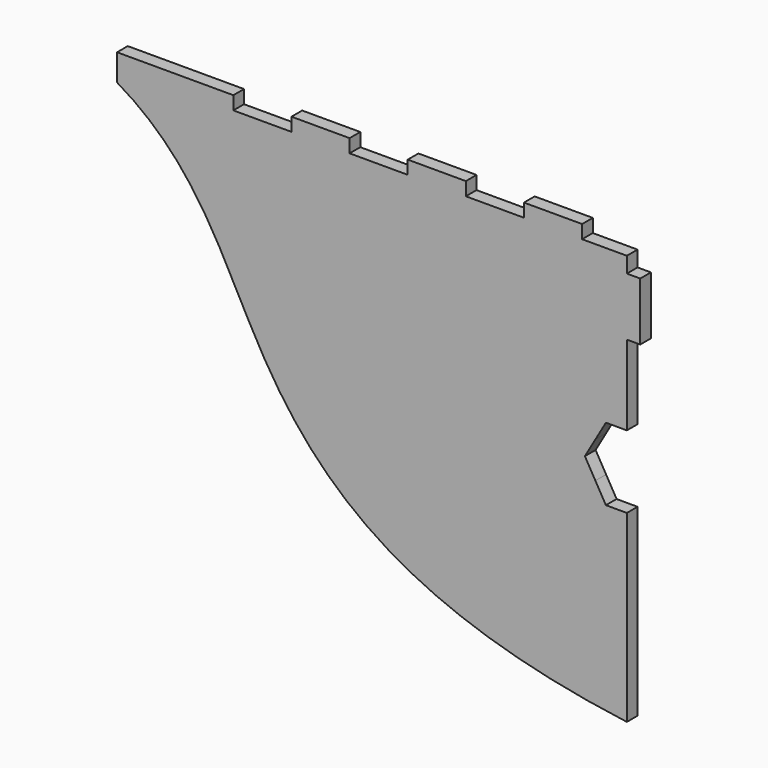
from build123d import *

# Parameters (mm, degrees)
F0_W      = 279.4
F0_H      = 330.2
F1_DEPTH  = 5.842
F2_W      = 25.4
F2_H      = 5.842
F2_W_2    = 76.2
F2_W_3    = 5.842
F2_H_2    = 25.4
F2_H_3    = 38.1
F3_DEPTH  = 5.842
F5_W      = 5.842
F5_H      = 12.7
F6_DEPTH  = 5.842
F7_DEPTH  = 5.842
F8_W      = 5.842
F8_H      = 25.4
F8_H_2    = 48.641
F8_H_3    = 34.925
F8_H_4    = 11.684
F9_DEPTH  = 5.842
F10_W     = 246.7240431406
F10_H     = 1.016
F11_DEPTH = 5.842
F13_W     = 25.4
F13_H     = 5.842
F13_W_2   = 19.558
F14_DEPTH = 5.842


# Not quite as in the source:
# - a feature names something its author has since deleted; it is built from what else it names


with BuildPart() as f1:
    # F0 (on Front) → F1 (new body)
    with BuildSketch(Plane.XZ):
        with Locations((25.751306051, 40.8756073241)):
            Rectangle(F0_W, F0_H)
    extrude(amount=F1_DEPTH)

    # F2 (on face) → F3 (cut, through all)
    with BuildSketch(Plane.XZ.offset(5.842)):
        with Locations((152.751306051, -121.3033926759)):
            Rectangle(F2_W, F2_H)
        with Locations((101.951306051, -121.3033926759)):
            Rectangle(F2_W, F2_H)
        with Locations((51.151306051, -121.3033926759)):
            Rectangle(F2_W, F2_H)
        with Locations((0.351306051, -121.3033926759)):
            Rectangle(F2_W, F2_H)
        with Locations((-75.848693949, -121.3033926759)):
            Rectangle(F2_W_2, F2_H)
        with Locations((162.530306051, -86.1243926759)):
            Rectangle(F2_W_3, F2_H_2)
        with Locations((162.530306051, -28.9743926759)):
            Rectangle(F2_W_3, F2_H_3)
        with Locations((-111.027693949, -86.1243926759)):
            Rectangle(F2_W_3, F2_H_2)
        with Locations((-111.027693949, -35.3243926759)):
            Rectangle(F2_W_3, F2_H_2)
        with Locations((-111.027693949, 15.4756073241)):
            Rectangle(F2_W_3, F2_H_2)
        with Locations((-111.027693949, 66.2756073241)):
            Rectangle(F2_W_3, F2_H_2)
        with Locations((-111.027693949, 167.8756073241)):
            Rectangle(F2_W_3, F2_H_2)
        with Locations((-111.027693949, 117.0756073241)):
            Rectangle(F2_W_3, F2_H_2)
    extrude(amount=-F3_DEPTH, mode=Mode.SUBTRACT)

    # F5 (on face) → F6 (cut, through all)
    with BuildSketch(Plane.XZ.offset(5.842)):
        with Locations((162.530306051, 2.7756073241)):
            Rectangle(F5_W, F5_H)
    extrude(amount=-F6_DEPTH, mode=Mode.SUBTRACT)

    # F4 (on face) → F7 (cut, through all)
    with BuildSketch(Plane.XZ.offset(5.842)):
        with BuildLine():
            Line((165.451306051, 15.4756073241), (159.609306051, 15.4756073241))
            add(Edge.make_bspline(
                [(159.609306051, 15.4756073241), (73.376306051, 28.1756073241), (-24.3765935073, 60.3637718481), (-21.873693949, 193.2756073241), (-113.948693949, 205.9756073241)],
                knots=[0, 0, 0, 0, 0.507272, 1, 1, 1, 1], degree=3))
            Line((-113.948693949, 205.9756073241), (-113.948693949, 180.5756073241))
            Line((-113.948693949, 180.5756073241), (-108.106693949, 180.5756073241))
            Line((-108.106693949, 180.5756073241), (-108.106693949, 155.1756073241))
            Line((-108.106693949, 155.1756073241), (-113.948693949, 155.1756073241))
            Line((-113.948693949, 155.1756073241), (-113.948693949, 129.7756073241))
            Line((-113.948693949, 129.7756073241), (-108.106693949, 129.7756073241))
            Line((-108.106693949, 129.7756073241), (-108.106693949, 104.3756073241))
            Line((-108.106693949, 104.3756073241), (-113.948693949, 104.3756073241))
            Line((-113.948693949, 104.3756073241), (-113.948693949, 78.9756073241))
            Line((-113.948693949, 78.9756073241), (-108.106693949, 78.9756073241))
            Line((-108.106693949, 78.9756073241), (-108.106693949, 53.5756073241))
            Line((-108.106693949, 53.5756073241), (-113.948693949, 53.5756073241))
            Line((-113.948693949, 53.5756073241), (-113.948693949, 28.1756073241))
            Line((-113.948693949, 28.1756073241), (-108.106693949, 28.1756073241))
            Line((-108.106693949, 28.1756073241), (-108.106693949, 2.7756073241))
            Line((-108.106693949, 2.7756073241), (-113.948693949, 2.7756073241))
            Line((-113.948693949, 2.7756073241), (-113.948693949, -22.6243926759))
            Line((-113.948693949, -22.6243926759), (-108.106693949, -22.6243926759))
            Line((-108.106693949, -22.6243926759), (-108.106693949, -48.0243926759))
            Line((-108.106693949, -48.0243926759), (-113.948693949, -48.0243926759))
            Line((-113.948693949, -48.0243926759), (-113.948693949, -73.4243926759))
            Line((-113.948693949, -73.4243926759), (-108.106693949, -73.4243926759))
            Line((-108.106693949, -73.4243926759), (-108.106693949, -98.8243926759))
            Line((-108.106693949, -98.8243926759), (-113.948693949, -98.8243926759))
            Line((-113.948693949, -98.8243926759), (-113.948693949, -118.3823926759))
            Line((-113.948693949, -118.3823926759), (-37.748693949, -118.3823926759))
            Line((-37.748693949, -118.3823926759), (-37.748693949, -124.2243926759))
            Line((-37.748693949, -124.2243926759), (-12.348693949, -124.2243926759))
            Line((-12.348693949, -124.2243926759), (-12.348693949, -118.3823926759))
            Line((-12.348693949, -118.3823926759), (13.051306051, -118.3823926759))
            Line((13.051306051, -118.3823926759), (13.051306051, -124.2243926759))
            Line((13.051306051, -124.2243926759), (38.451306051, -124.2243926759))
            Line((38.451306051, -124.2243926759), (38.451306051, -118.3823926759))
            Line((38.451306051, -118.3823926759), (63.851306051, -118.3823926759))
            Line((63.851306051, -118.3823926759), (63.851306051, -124.2243926759))
            Line((63.851306051, -124.2243926759), (89.251306051, -124.2243926759))
            Line((89.251306051, -124.2243926759), (89.251306051, -118.3823926759))
            Line((89.251306051, -118.3823926759), (114.651306051, -118.3823926759))
            Line((114.651306051, -118.3823926759), (114.651306051, -124.2243926759))
            Line((114.651306051, -124.2243926759), (140.051306051, -124.2243926759))
            Line((140.051306051, -124.2243926759), (140.051306051, -118.3823926759))
            Line((140.051306051, -118.3823926759), (165.451306051, -118.3823926759))
            Line((165.451306051, -118.3823926759), (165.451306051, -98.8243926759))
            Line((165.451306051, -98.8243926759), (159.609306051, -98.8243926759))
            Line((159.609306051, -98.8243926759), (159.609306051, -73.4243926759))
            Line((159.609306051, -73.4243926759), (165.451306051, -73.4243926759))
            Line((165.451306051, -73.4243926759), (165.451306051, -48.0243926759))
            Line((165.451306051, -48.0243926759), (159.609306051, -48.0243926759))
            Line((159.609306051, -48.0243926759), (159.609306051, -9.9243926759))
            Line((159.609306051, -9.9243926759), (165.451306051, -9.9243926759))
            Line((165.451306051, -9.9243926759), (165.451306051, 15.4756073241))
        make_face()
        with BuildLine():
            add(Edge.make_bspline(
                [(159.609306051, 15.4756073241), (73.376306051, 28.1756073241), (-24.3765935073, 60.3637718481), (-21.873693949, 193.2756073241), (-113.948693949, 205.9756073241)],
                knots=[0, 0, 0, 0, 0.507272, 1, 1, 1, 1], degree=3))
            Line((159.609306051, 15.4756073241), (159.609306051, 21.8256073241))
            add(Edge.make_bspline(
                [(159.609306051, 21.8256073241), (63.851306051, 34.5256073241), (-5.6173037023, 95.4914607938), (-31.4644745687, 187.7697107475), (-87.114737086, 205.9756073241)],
                knots=[0, 0, 0, 0, 0.5236819738, 0.940243193, 0.940243193, 0.940243193, 0.940243193], degree=3))
            Line((-87.114737086, 205.9756073241), (-113.948693949, 205.9756073241))
        make_face()
    extrude(amount=-F7_DEPTH, mode=Mode.SUBTRACT)

    # F8 (on face) → F9 (cut, through all)
    with BuildSketch(Plane.XZ.offset(5.842)):
        Polygon((165.451306051, 15.4756073241), (165.451306051, 28.1756073241), (159.609306051, 28.1756073241), (159.609306051, 21.8256073241), (159.609306051, 15.4756073241), align=None)
        with Locations((162.530306051, 40.8756073241)):
            Rectangle(F8_W, F8_H)
        with Locations((162.530306051, 77.8961073241)):
            Rectangle(F8_W, F8_H_2)
        with BuildLine():
            Line((159.609306051, 102.2166073241), (165.451306051, 102.2166073241))
            Line((165.451306051, 102.2166073241), (165.451306051, 103.3306229057))
            ThreePointArc((165.451306051, 103.3306229057), (162.5829399691, 102.4975980153), (159.609306051, 102.2166073241))
        make_face()
        with BuildLine():
            ThreePointArc((145.861152343, 110.1541080567), (151.6718056847, 104.3434542505), (159.609306051, 102.2166073241))
            Line((159.609306051, 102.2166073241), (159.609306051, 133.9666073241))
            ThreePointArc((159.609306051, 133.9666073241), (151.6718056847, 131.8397603977), (145.861152343, 126.0291065915))
            ThreePointArc((145.861152343, 126.0291065915), (143.734306051, 118.0916073241), (145.861152343, 110.1541080567))
        make_face()
        with BuildLine():
            Line((150.4438705276, 102.2166073241), (159.609306051, 102.2166073241))
            ThreePointArc((159.609306051, 102.2166073241), (151.6718056847, 104.3434542505), (145.861152343, 110.1541080567))
            Line((145.861152343, 110.1541080567), (150.4438705276, 102.2166073241))
        make_face()
        with BuildLine():
            Line((159.609306051, 133.9666073241), (159.609306051, 102.2166073241))
            ThreePointArc((159.609306051, 102.2166073241), (162.5829399691, 102.4975980153), (165.451306051, 103.3306229057))
            Line((165.451306051, 103.3306229057), (165.451306051, 132.8525917425))
            ThreePointArc((165.451306051, 132.8525917425), (162.5829399691, 133.6856166328), (159.609306051, 133.9666073241))
        make_face()
        with BuildLine():
            Line((165.451306051, 133.9666073241), (159.609306051, 133.9666073241))
            ThreePointArc((159.609306051, 133.9666073241), (162.5829399691, 133.6856166328), (165.451306051, 132.8525917425))
            Line((165.451306051, 132.8525917425), (165.451306051, 133.9666073241))
        make_face()
        with BuildLine():
            ThreePointArc((145.861152343, 126.0291065915), (151.6718056847, 131.8397603977), (159.609306051, 133.9666073241))
            Line((159.609306051, 133.9666073241), (150.4438705276, 133.9666073241))
            Line((150.4438705276, 133.9666073241), (145.861152343, 126.0291065915))
        make_face()
        with Locations((162.530306051, 151.4291073241)):
            Rectangle(F8_W, F8_H_3)
        with BuildLine():
            Line((141.2784350042, 118.0916073241), (145.861152343, 110.1541080567))
            ThreePointArc((145.861152343, 110.1541080567), (143.734306051, 118.0916073241), (145.861152343, 126.0291065915))
            Line((145.861152343, 126.0291065915), (141.2784350042, 118.0916073241))
        make_face()
        with Locations((162.530306051, 200.1336073241)):
            Rectangle(F8_W, F8_H_4)
    extrude(amount=-F9_DEPTH, mode=Mode.SUBTRACT)

    # F10 (on face) → F11 (join, through all)
    with BuildSketch(Plane.XZ.offset(5.842)):
        with Locations((36.2472844807, 206.4836073241)):
            Rectangle(F10_W, F10_H)
    extrude(amount=-F11_DEPTH)

    # F13 (on face) → F14 (cut, through all)
    with BuildSketch(Plane.XZ.offset(5.842)):
        with Locations((51.151306051, 204.0706073241)):
            Rectangle(F13_W, F13_H)
        with Locations((101.951306051, 204.0706073241)):
            Rectangle(F13_W, F13_H)
        with Locations((149.830306051, 204.0706073241)):
            Rectangle(F13_W_2, F13_H)
        with BuildLine():
            add(Edge.make_bspline(
                [(-64.0656111495, 195.8912068503), (-64.4986133811, 197.8821506555), (-64.5462177809, 200.9608220943), (-64.8897370896, 206.9916073241)],
                knots=[0.7783755915, 0.7783755915, 0.7783755915, 0.7783755915, 1, 1, 1, 1], degree=3))
            Line((-64.8897370896, 206.9916073241), (-87.1147370896, 206.9916073241))
            Line((-87.1147370896, 206.9916073241), (-87.1147370896, 205.9756073241))
            add(Edge.make_bspline(
                [(-64.0656111419, 195.8912068549), (-70.8038372609, 199.7329606353), (-78.4197996839, 203.1310721158), (-87.114737086, 205.9756073241)],
                knots=[0.8751586172, 0.8751586172, 0.8751586172, 0.8751586172, 0.940243193, 0.940243193, 0.940243193, 0.940243193], degree=3))
        make_face()
        with Locations((0.351306051, 204.0706073241)):
            Rectangle(F13_W, F13_H)
        with BuildLine():
            Line((-63.148693949, 195.362557311), (-63.148693949, 206.9916073241))
            Line((-63.148693949, 206.9916073241), (-64.8897370896, 206.9916073241))
            add(Edge.make_bspline(
                [(-64.0656111495, 195.8912068503), (-64.4986133811, 197.8821506555), (-64.5462177809, 200.9608220943), (-64.8897370896, 206.9916073241)],
                knots=[0.7783755915, 0.7783755915, 0.7783755915, 0.7783755915, 1, 1, 1, 1], degree=3))
            add(Edge.make_bspline(
                [(-63.148693949, 195.362557311), (-63.4525182871, 195.5396905387), (-63.7581509788, 195.7159105346), (-64.0656111419, 195.8912068549)],
                knots=[0.8721888572, 0.8721888572, 0.8721888572, 0.8721888572, 0.8751586172, 0.8751586172, 0.8751586172, 0.8751586172], degree=3))
        make_face()
    extrude(amount=-F14_DEPTH, mode=Mode.SUBTRACT)


solid = f1.part
